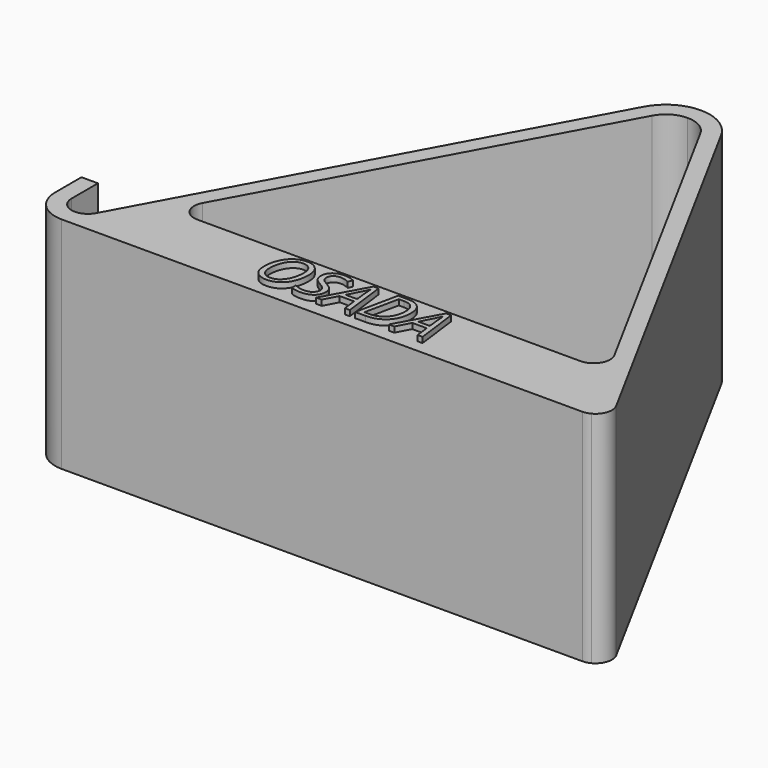
from build123d import *

# Parameters (mm, degrees)
F1_DEPTH     = 40
F2_TEXT_SIZE = 10.8333333628
F3_DEPTH     = 1


# Not quite as in the source:
# - Text() gives the source's letters only with a copy of the font that has no kerning and outlines rounded to 1/6400 em; it was checked with that copy


with BuildPart() as f1:
    # F0 (on Top) → F1 (new body)
    with BuildSketch(Plane.XY):
        with BuildLine():
            Line((0, -6), (50, -6))
            Line((50, -6), (94.8015433725, -6))
            ThreePointArc((94.8015433725, -6), (95.5402940463, -5.9076188612), (96.2335469677, -5.6361649613))
            ThreePointArc((96.2335469677, -5.6361649613), (97.6781729458, -3.8514706677), (97.4377083338, -1.5679964048))
            Line((97.4377083338, -1.5679964048), (57.0297732302, 72.8186762538))
            ThreePointArc((57.0297732302, 72.8186762538), (50, 77), (42.9702267698, 72.8186762538))
            Line((42.9702267698, 72.8186762538), (2.6361649613, -1.4320035952))
            ThreePointArc((2.6361649613, -1.4320035952), (1.5336214028, -2.5783726249), (0, -3))
            ThreePointArc((0, -3), (-2.0506106437, -2.1506092602), (-2.9000013835, -0.0999986165))
            Line((-2.9000013835, -0.0999986165), (-2.9000013835, 5.9000013835))
            Line((-2.9000013835, 5.9000013835), (-5.9000013835, 5.9000013835))
            Line((-5.9000013835, 5.9000013835), (-5.9000013835, -0.0999986165))
            ThreePointArc((-5.9000013835, -0.0999986165), (-4.1719309873, -4.2719296038), (0, -6))
        make_face()
        with BuildLine():
            ThreePointArc((50, 74), (52.5560356714, 73.2972877081), (54.3936082689, 71.3866726586))
            Line((54.3936082689, 71.3866726586), (87.5050813829, 10.4320035952))
            ThreePointArc((87.5050813829, 10.4320035952), (87.4472890465, 7.4663785972), (84.8689164216, 6))
            Line((84.8689164216, 6), (50, 6))
            Line((50, 6), (15.1310835784, 6))
            ThreePointArc((15.1310835784, 6), (12.5527109535, 7.4663785972), (12.4949186171, 10.4320035952))
            Line((12.4949186171, 10.4320035952), (45.6063917311, 71.3866726586))
            ThreePointArc((45.6063917311, 71.3866726586), (47.4439643286, 73.2972877081), (50, 74))
        make_face(mode=Mode.SUBTRACT)
    extrude(amount=F1_DEPTH)

    # F2 (on face) → F3 (join)
    with BuildSketch(Plane.XY.offset(40)):
        with Locations((31.9007635117, -3.7000016309)):
            Text('OSADA', F2_TEXT_SIZE, font='Open Sans', font_style=FontStyle.ITALIC, text_align=(TextAlign.LEFT, TextAlign.BOTTOM))
    extrude(amount=F3_DEPTH)


solid = f1.part
